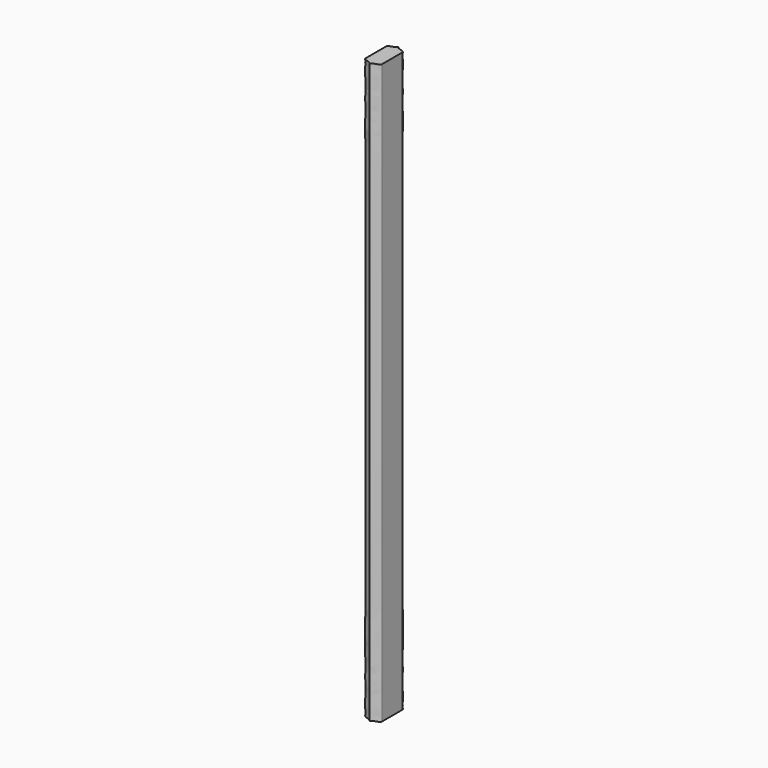
from build123d import *

# Parameters (mm, degrees)
F2_DEPTH = 1600


# Not quite as in the source:
# - a feature of the source that left no trace in its solid (it failed there, or was rolled back) is left out


with BuildPart() as f2:
    # F0 (on Top) → F2 (new body)
    with BuildSketch(Plane.XY):
        with BuildLine():
            add(Edge.make_bspline(
                [(50, 0), (50, 7), (27.5, 7), (27.5, 14.625)],
                knots=[0, 0, 0, 0, 26.8354359942, 26.8354359942, 26.8354359942, 26.8354359942], degree=3))
            add(Edge.make_bspline(
                [(50, 0), (50, 7), (72.5, 7), (72.5, 14.625)],
                knots=[0, 0, 0, 0, 26.8354359942, 26.8354359942, 26.8354359942, 26.8354359942], degree=3))
            Line((72.5, 14.625), (72.5, 85.375))
            add(Edge.make_bspline(
                [(50, 100), (50, 93), (72.5, 93), (72.5, 85.375)],
                knots=[0, 0, 0, 0, 26.8354359942, 26.8354359942, 26.8354359942, 26.8354359942], degree=3))
            add(Edge.make_bspline(
                [(50, 100), (50, 93), (27.5, 93), (27.5, 85.375)],
                knots=[0, 0, 0, 0, 26.8354359942, 26.8354359942, 26.8354359942, 26.8354359942], degree=3))
            Line((27.5, 85.375), (27.5, 14.625))
        make_face()
    extrude(amount=F2_DEPTH)


solid = f2.part
